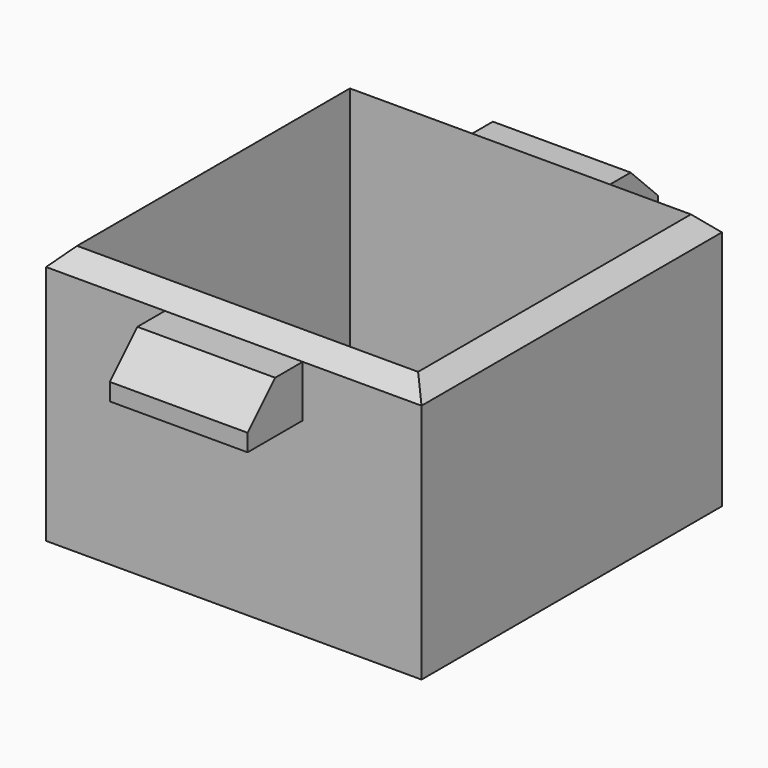
from build123d import *

# Parameters (mm, degrees)
F0_W         = 54.5
F0_H         = 20
F1_DEPTH     = 54.5
F2_DEPTH     = 20
F3_T         = -2.5
F4_W         = 10
F4_H         = 7.5
F5_DEPTH     = 10
F6_W         = 10
F6_H         = 7.5
F7_DEPTH     = 10
F8_T1_DEPTH  = 45.7168298797
F8_T3_DEPTH  = 80.2168298797
F8_T8_DEPTH  = 80.2168298797
F8_T14_DEPTH = 80.2168298797
F8_T21_DEPTH = 80.2168298797
F8_T27_DEPTH = 80.2168298797
F8_T33_DEPTH = 80.2168298797
F8_T40_DEPTH = 80.2168298797


# Not quite as in the source:
# - a fillet or chamfer that OpenCascade refuses, or shapes differently, is made with other operations: its cross-section is extruded or revolved along the edge and cut away or added


with BuildPart() as f1:
    # F0 (on Front) → F1 (new body)
    with BuildSketch(Plane.XZ):
        Rectangle(F0_W, F0_H)
    extrude(amount=F1_DEPTH)

    # F2 (add): a face of the model
    f2_faces = [f1.faces().sort_by_distance(p)[0] for p in [
        (0, -27.25, 10),
    ]]
    extrude(f2_faces, amount=F2_DEPTH)

    # F3
    f3_openings = [f1.faces().sort_by_distance(p)[0] for p in [
        (0, -27.25, 30),
    ]]
    offset(amount=F3_T, openings=f3_openings)

    # F4 (on face) → F5 (join)
    with BuildSketch(Plane.XZ.offset(54.5)):
        with Locations((-5, 21.25)):
            Rectangle(F4_W, F4_H)
        with Locations((5, 21.25)):
            Rectangle(F4_W, F4_H)
    extrude(amount=F5_DEPTH)

    # F6 (on face) → F7 (join)
    with BuildSketch(Plane(origin=(0, 0, 0), x_dir=(-1, 0, 0), z_dir=(0, 1, 0))):
        with Locations((-5, 21.25)):
            Rectangle(F6_W, F6_H)
        with Locations((5, 21.25)):
            Rectangle(F6_W, F6_H)
    extrude(amount=F7_DEPTH)

    # F8: chamfer of 5 on 6 edges, made by hand

    # F8_s2 → F8_t1 (cut)
    with BuildSketch(Plane.YZ.offset(-22.8584149398)):
        Polygon((5, 25), (10, 20), (10, 25), align=None)
        Polygon((-59.5, 25), (-64.5, 20), (-64.5, 25), align=None)
    extrude(amount=F8_T1_DEPTH, mode=Mode.SUBTRACT)

    # F8_s4 → F8_t3 (cut)
    with BuildSketch(Plane.XZ.offset(-12.8584149398)):
        Polygon((-22.25, 30), (-27.25, 25), (-27.25, 30), align=None)
        Polygon((27.25, 25), (22.25, 30), (27.25, 30), align=None)
    extrude(amount=F8_T3_DEPTH, mode=Mode.SUBTRACT)


with BuildPart() as f8_tool6:
    # F8_s7 → F8_t8 (new body)
    with BuildSketch(Plane.YZ.offset(40.1084149398)):
        Polygon((-5, 30), (0, 25), (0, 30), align=None)
    extrude(amount=-F8_T8_DEPTH)

    split(bisect_by=Plane.YZ.offset(10), keep=Keep.TOP)

    split(bisect_by=Plane.XY.offset(25), keep=Keep.TOP)


with BuildPart() as f1_1:
    add(f1.part)

    # F8_t5: cut F8_tool6
    add(f8_tool6.part, mode=Mode.SUBTRACT)


with BuildPart() as f8_tool12:
    # F8_s13 → F8_t14 (new body)
    with BuildSketch(Plane.YZ.offset(40.1084149398)):
        Polygon((-5, 30), (0, 25), (0, 30), align=None)
    extrude(amount=-F8_T14_DEPTH)

    split(bisect_by=Plane.YZ.offset(10), keep=Keep.BOTTOM)

    split(bisect_by=Plane.XY.offset(25), keep=Keep.TOP)

    split(bisect_by=Plane.YZ.offset(-10), keep=Keep.TOP)


with BuildPart() as f1_2:
    add(f1_1.part)

    # F8_t11: cut F8_tool12
    add(f8_tool12.part, mode=Mode.SUBTRACT)


with BuildPart() as f8_tool19:
    # F8_s20 → F8_t21 (new body)
    with BuildSketch(Plane.YZ.offset(40.1084149398)):
        Polygon((-5, 30), (0, 25), (0, 30), align=None)
    extrude(amount=-F8_T21_DEPTH)

    split(bisect_by=Plane.XY.offset(25), keep=Keep.TOP)

    split(bisect_by=Plane.YZ.offset(-10), keep=Keep.BOTTOM)


with BuildPart() as f1_3:
    add(f1_2.part)

    # F8_t18: cut F8_tool19
    add(f8_tool19.part, mode=Mode.SUBTRACT)


with BuildPart() as f8_tool25:
    # F8_s26 → F8_t27 (new body)
    with BuildSketch(Plane.YZ.offset(40.1084149398)):
        Polygon((-54.5, 25), (-49.5, 30), (-54.5, 30), align=None)
    extrude(amount=-F8_T27_DEPTH)

    split(bisect_by=Plane.YZ.offset(10), keep=Keep.TOP)

    split(bisect_by=Plane.XY.offset(25), keep=Keep.TOP)


with BuildPart() as f1_4:
    add(f1_3.part)

    # F8_t24: cut F8_tool25
    add(f8_tool25.part, mode=Mode.SUBTRACT)


with BuildPart() as f8_tool31:
    # F8_s32 → F8_t33 (new body)
    with BuildSketch(Plane.YZ.offset(40.1084149398)):
        Polygon((-54.5, 25), (-49.5, 30), (-54.5, 30), align=None)
    extrude(amount=-F8_T33_DEPTH)

    split(bisect_by=Plane.YZ.offset(-10), keep=Keep.TOP)

    split(bisect_by=Plane.YZ.offset(10), keep=Keep.BOTTOM)

    split(bisect_by=Plane.XY.offset(25), keep=Keep.TOP)


with BuildPart() as f1_5:
    add(f1_4.part)

    # F8_t30: cut F8_tool31
    add(f8_tool31.part, mode=Mode.SUBTRACT)


with BuildPart() as f8_tool38:
    # F8_s39 → F8_t40 (new body)
    with BuildSketch(Plane.YZ.offset(40.1084149398)):
        Polygon((-54.5, 25), (-49.5, 30), (-54.5, 30), align=None)
    extrude(amount=-F8_T40_DEPTH)

    split(bisect_by=Plane.YZ.offset(-10), keep=Keep.BOTTOM)

    split(bisect_by=Plane.XY.offset(25), keep=Keep.TOP)


with BuildPart() as f1_6:
    add(f1_5.part)

    # F8_t37: cut F8_tool38
    add(f8_tool38.part, mode=Mode.SUBTRACT)


solid = f1_6.part
